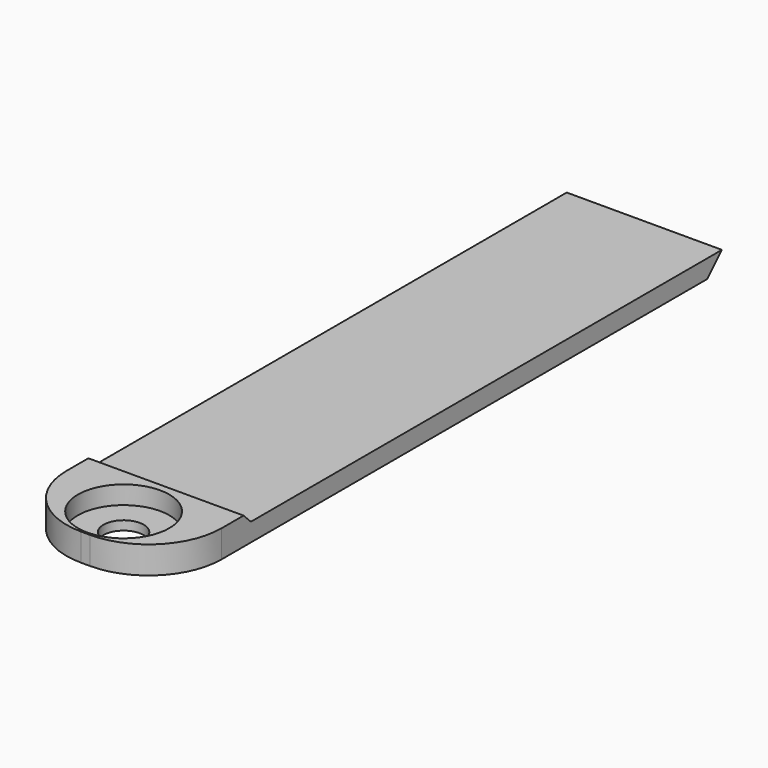
from build123d import *

# Parameters (mm, degrees)
F0_W     = 17
F0_H     = 64.5
F0_H_2   = 12
F0_R     = 5
F1_DEPTH = 2
F2_R     = 8
F3_SIZE  = 1.99999
F0_R_2   = 2.2
F4_DEPTH = 1
F5_DEPTH = 3
F6_R     = 8
F7_SIZE  = 0.99999


# Not quite as in the source:
# - a fillet or chamfer is up to 0.001 mm smaller than in the source, because OpenCascade refuses the exact size


with BuildPart() as f1:
    # F0 (on Top) → F1 (new body)
    with BuildSketch(Plane.XY):
        with Locations((0, 6)):
            Rectangle(F0_W, F0_H)
        with Locations((0, -32.25)):
            Rectangle(F0_W, F0_H_2)
        with Locations((0, -33.05)):
            Circle(F0_R, mode=Mode.SUBTRACT)
    extrude(amount=F1_DEPTH)

    # F2
    f2_edges = [f1.edges().sort_by_distance(p)[0] for p in [
        (8.5, -38.25, 1),
        (-8.5, -38.25, 1),
    ]]
    fillet(f2_edges, radius=F2_R)

    # F3 (size 2 in the source; OpenCascade refuses exactly that, so slightly less here)
    f3_edges = [f1.edges().sort_by_distance(p)[0] for p in [
        (0, 38.25, 0),
    ]]
    chamfer(f3_edges, length=F3_SIZE)

    # F0 (on Top) → F4 (join)
    with BuildSketch(Plane.XY):
        with Locations((0, -33.05)):
            Circle(F0_R)
        with Locations((0, -33.05)):
            Circle(F0_R_2, mode=Mode.SUBTRACT)
    extrude(amount=F4_DEPTH)

    # F0 (on Top) → F5 (join)
    with BuildSketch(Plane.XY):
        with Locations((0, -32.25)):
            Rectangle(F0_W, F0_H_2)
        with Locations((0, -33.05)):
            Circle(F0_R, mode=Mode.SUBTRACT)
    extrude(amount=F5_DEPTH)

    # F6
    f6_edges = [f1.edges().sort_by_distance(p)[0] for p in [
        (8.5, -38.25, 1.5),
        (-8.5, -38.25, 1.5),
    ]]
    fillet(f6_edges, radius=F6_R)

    # F7 (size 1 in the source; OpenCascade refuses exactly that, so slightly less here)
    f7_edges = [f1.edges().sort_by_distance(p)[0] for p in [
        (0, -26.25, 3),
    ]]
    chamfer(f7_edges, length=F7_SIZE)


solid = f1.part
